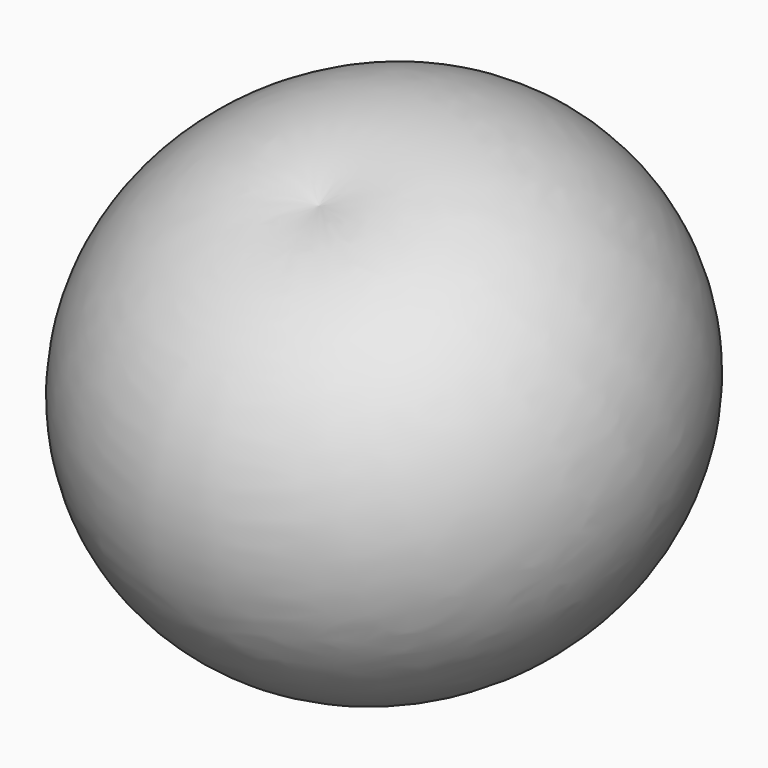
from build123d import *
from build123d import SkipClean  # not in build123d's __all__


with BuildPart() as f1:
    # F0 (on Right) → F1 (revolve)
    with BuildSketch(Plane.YZ):
        with BuildLine():
            add(Edge.make_bspline(
                [(40.8417056283, -29.8455245679), (37.35877147, -28.4480000079), (32.8929983079, -28.4480000079)],
                knots=[0.8945338201, 0.8945338201, 0.8945338201, 1.5707963268, 1.5707963268, 1.5707963268], degree=2, weights=[1, 0.9433762219, 1]))
            add(Edge.make_bspline(
                [(42.105613437, -30.4271384657), (41.5130824533, -30.1149139847), (40.8417056283, -29.8455245679)],
                knots=[0.7591769731, 0.7591769731, 0.7591769731, 0.8945338201, 0.8945338201, 0.8945338201], degree=2, weights=[1, 0.9977106895, 1]))
            ThreePointArc((42.105613437, -30.4271384657), (44.0714983156, -5.1881798652), (18.9229976386, -2.2859999444))
            Line((18.9229976386, -2.2859999444), (30.2253543952, -28.589665369))
            add(Edge.make_bspline(
                [(32.8929983079, -28.4480000079), (31.5441300596, -28.4480000079), (30.2253543952, -28.589665369)],
                knots=[1.5707963268, 1.5707963268, 1.5707963268, 1.782423145, 1.782423145, 1.782423145], degree=2, weights=[1, 0.9944069827, 1]))
        make_face()
    revolve(axis=Axis((0, 25.9079979733, -18.5419999762), (0, 0.3947854392, -0.9187733436)))

    # F0 (on Right) → F2 (revolve)
    with BuildSketch(Plane.YZ):
        with BuildLine():
            add(Edge.make_bspline(
                [(40.8417056283, -29.8455245679), (41.1604426392, -30.1623492327), (41.4435980593, -30.4745855709), (41.6942473899, -30.7816924182)],
                knots=[0, 0, 0, 0, 0.0255071894, 0.0255071894, 0.0255071894, 0.0255071894], degree=3))
            add(Edge.make_bspline(
                [(40.8417056283, -29.8455245679), (37.35877147, -28.4480000079), (32.8929983079, -28.4480000079)],
                knots=[0.8945338201, 0.8945338201, 0.8945338201, 1.5707963268, 1.5707963268, 1.5707963268], degree=2, weights=[1, 0.9433762219, 1]))
            Line((32.8929983079, -28.4480000079), (32.8929983079, -34.7980000079))
            Line((32.8929983079, -34.7980000079), (32.8929983079, -40.6381264329))
            add(Edge.make_bspline(
                [(41.6942473899, -30.7816924182), (44.6618466499, -34.4177286711), (42.3020218601, -38.7497275544), (40.7608179336, -39.7736108081), (38.7694217239, -40.3810728072), (36.8220473508, -40.7352669513), (34.3392785671, -40.673359824), (32.8929983079, -40.6381264329)],
                knots=[0.0255071894, 0.0255071894, 0.0255071894, 0.0255071894, 0.3275032737, 0.4739978855, 0.6255118689, 0.7806480871, 1, 1, 1, 1], degree=3))
        make_face()
    with SkipClean():  # cleaning this boolean's faces spoils the solid; the shape is the same uncleaned
        revolve(axis=Axis((0, 32.8929983079, -34.7980000079), (0, 0, -1)))


solid = f1.part
